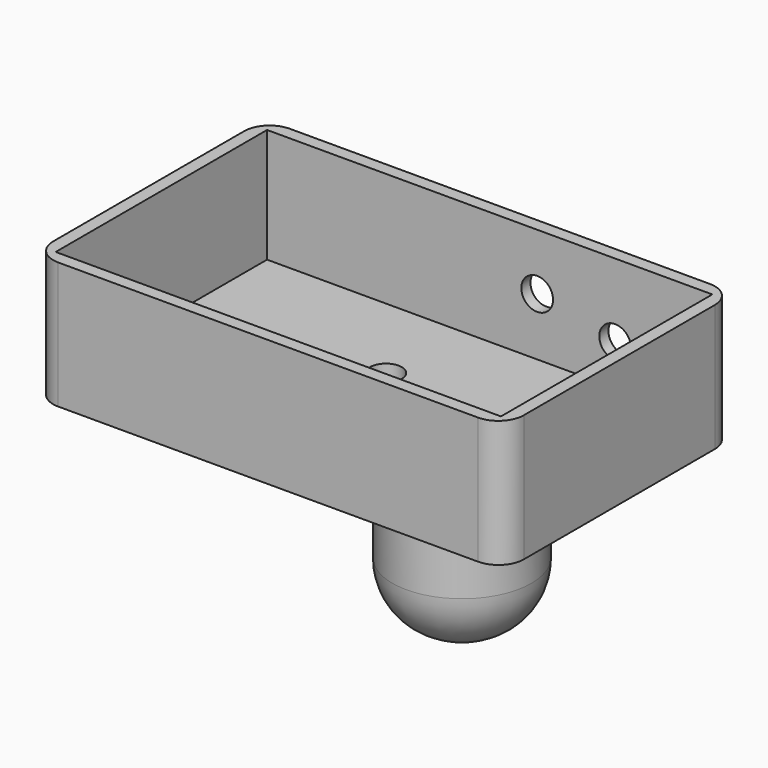
from build123d import *

# Parameters (mm, degrees)
F0_W           = 94.2332278937
F0_H           = 57.9777825624
F1_DEPTH       = 25.4
F2_T           = -2.54
F3_R           = 5.08
F5_D           = 6.35
F7_D           = 6.35
F7_DEPTH       = 12.7
F7_CBORE_D     = 12.7
F7_CBORE_DEPTH = 0.254
F7_TIP         = 1.9077324654
F9_D           = 6.35
F9_DEPTH       = 12.7
F9_CBORE_D     = 12.7
F9_CBORE_DEPTH = 0.254
F9_TIP         = 1.9077324654
F10_R          = 13.9169366501
F11_DEPTH      = 25.4
F12_R          = 12.7
F13_W          = 27.7714207768
F13_H          = 7.534484379
F14_DEPTH      = 25.4
F15_R          = 12.7
F16_T1_DEPTH   = 12.7
F16_T3_DEPTH   = 2.3714207768
F16_T6_ANGLE   = 90
F16_T8_ANGLE   = 90
F16_T10_ANGLE  = 90
F16_T12_ANGLE  = 90


# Not quite as in the source:
# - a fillet or chamfer that OpenCascade refuses, or shapes differently, is made with other operations: its cross-section is extruded or revolved along the edge and cut away or added


with BuildPart() as f1:
    # F0 (on Top) → F1 (new body)
    with BuildSketch(Plane.XY):
        with Locations((-38.147569634, 3.4275231883)):
            Rectangle(F0_W, F0_H)
    extrude(amount=F1_DEPTH)

    # F2
    f2_openings = [f1.faces().sort_by_distance(p)[0] for p in [
        (-38.14757, 3.427523, 25.4),
    ]]
    offset(amount=F2_T, openings=f2_openings)

    # F3
    f3_edges = [f1.edges().sort_by_distance(p)[0] for p in [
        (-85.264184, -25.561368, 12.7),
        (8.969044, -25.561368, 12.7),
        (8.969044, 32.416414, 12.7),
        (-85.264184, 32.416414, 12.7),
    ]]
    fillet(f3_edges, radius=F3_R)

    # F5 (through all)
    with Locations(Plane.XY.offset(2.54)):
        with Locations((-44.2425459623, 11.5331579)):
            Hole(F5_D / 2)

    # F7
    with Locations(Plane.XY.offset(2.54)):
        with Locations((-63.0617812276, -7.2897328064)):
            CounterBoreHole(F7_D / 2, F7_CBORE_D / 2, F7_CBORE_DEPTH, depth=F7_DEPTH)
            with Locations((0, 0, -(F7_DEPTH + F7_TIP / 2))):  # 118° drill point
                Cone(0, F7_D / 2, F7_TIP, mode=Mode.SUBTRACT)

    # F9
    with Locations(Plane(origin=(0, 32.4164144695, 0), x_dir=(-1, 0, 0), z_dir=(0, 1, 0))):
        with Locations((13.0262067541, 10.6704961509), (28.6341179162, 14.0921706334)):
            CounterBoreHole(F9_D / 2, F9_CBORE_D / 2, F9_CBORE_DEPTH, depth=F9_DEPTH)
            with Locations((0, 0, -(F9_DEPTH + F9_TIP / 2))):  # 118° drill point
                Cone(0, F9_D / 2, F9_TIP, mode=Mode.SUBTRACT)

    # F10 (on face) → F11 (join)
    with BuildSketch(Plane(origin=(0, 0, 0), x_dir=(1, 0, 0), z_dir=(0, 0, -1))):
        with Locations((-14.1745125875, 7.0280302316)):
            Circle(F10_R)
    extrude(amount=F11_DEPTH)

    # F12
    f12_edges = [f1.edges().sort_by_distance(p)[0] for p in [
        (-28.091449, -7.02803, -25.4),
    ]]
    fillet(f12_edges, radius=F12_R)

    # F13 (on face) → F14 (join)
    with BuildSketch(Plane(origin=(0, 0, 0), x_dir=(1, 0, 0), z_dir=(0, 0, -1))):
        with Locations((-67.7874796093, -15.7441017218)):
            Rectangle(F13_W, F13_H)
    extrude(amount=F14_DEPTH)

    # F15
    f15_edges = [f1.edges().sort_by_distance(p)[0] for p in [
        (-53.901769, 15.744102, -25.4),
        (-81.67319, 15.744102, -25.4),
    ]]
    fillet(f15_edges, radius=F15_R)

    # F16: fillet of radius 5.08 on 2 edges, made by hand

    # F16_s2 → F16_t1 (cut)
    with BuildSketch(Plane.XY.offset(-12.7)):
        with BuildLine():
            ThreePointArc((-58.9817692208, 19.5113439113), (-55.3896667724, 18.0234463597), (-53.9017692208, 14.4313439113))
            Line((-53.9017692208, 14.4313439113), (-53.9017692208, 19.5113439113))
            Line((-53.9017692208, 19.5113439113), (-58.9817692208, 19.5113439113))
        make_face()
        with BuildLine():
            ThreePointArc((-81.6731899977, 14.4313439113), (-80.1852924461, 18.0234463597), (-76.5931899977, 19.5113439113))
            Line((-76.5931899977, 19.5113439113), (-81.6731899977, 19.5113439113))
            Line((-81.6731899977, 19.5113439113), (-81.6731899977, 14.4313439113))
        make_face()
        with BuildLine():
            ThreePointArc((-81.6731899977, 17.0568595323), (-80.1852924461, 13.4647570839), (-76.5931899977, 11.9768595323))
            Line((-76.5931899977, 11.9768595323), (-81.6731899977, 11.9768595323))
            Line((-81.6731899977, 11.9768595323), (-81.6731899977, 17.0568595323))
        make_face()
        with BuildLine():
            ThreePointArc((-58.9817692208, 11.9768595323), (-55.3896667724, 13.4647570839), (-53.9017692208, 17.0568595323))
            Line((-53.9017692208, 17.0568595323), (-53.9017692208, 11.9768595323))
            Line((-53.9017692208, 11.9768595323), (-58.9817692208, 11.9768595323))
        make_face()
    extrude(amount=F16_T1_DEPTH, mode=Mode.SUBTRACT)

    # F16_s4 → F16_t3 (cut)
    with BuildSketch(Plane.YZ.offset(-68.9731899977)):
        with BuildLine():
            ThreePointArc((19.5113439113, -20.32), (18.0234463597, -23.9121024484), (14.4313439113, -25.4))
            Line((14.4313439113, -25.4), (19.5113439113, -25.4))
            Line((19.5113439113, -25.4), (19.5113439113, -20.32))
        make_face()
        with BuildLine():
            ThreePointArc((11.9768595323, -20.32), (13.4647570839, -23.9121024484), (17.0568595323, -25.4))
            Line((17.0568595323, -25.4), (11.9768595323, -25.4))
            Line((11.9768595323, -25.4), (11.9768595323, -20.32))
        make_face()
    extrude(amount=F16_T3_DEPTH, mode=Mode.SUBTRACT)

    # F16_s5 → F16_t6 (revolve, cut)
    with BuildSketch(Plane.XY.offset(-12.7)):
        with BuildLine():
            ThreePointArc((-76.5931899977, 11.9768595323), (-80.1852924461, 13.4647570839), (-81.6731899977, 17.0568595323))
            Line((-81.6731899977, 17.0568595323), (-81.6731899977, 11.9768595323))
            Line((-81.6731899977, 11.9768595323), (-76.5931899977, 11.9768595323))
        make_face()
    revolve(axis=Axis((-68.9731899977, 11.9768595323, -12.7), (0, -1, 0)), revolution_arc=F16_T6_ANGLE, mode=Mode.SUBTRACT)

    # F16_s7 → F16_t8 (revolve, cut)
    with BuildSketch(Plane.XY.offset(-12.7)):
        with BuildLine():
            ThreePointArc((-58.9817692208, 19.5113439113), (-55.3896667724, 18.0234463597), (-53.9017692208, 14.4313439113))
            Line((-53.9017692208, 14.4313439113), (-53.9017692208, 19.5113439113))
            Line((-53.9017692208, 19.5113439113), (-58.9817692208, 19.5113439113))
        make_face()
    revolve(axis=Axis((-66.6017692208, 19.5113439113, -12.7), (0, 1, 0)), revolution_arc=F16_T8_ANGLE, mode=Mode.SUBTRACT)

    # F16_s9 → F16_t10 (revolve, cut)
    with BuildSketch(Plane.XY.offset(-12.7)):
        with BuildLine():
            ThreePointArc((-81.6731899977, 14.4313439113), (-80.1852924461, 18.0234463597), (-76.5931899977, 19.5113439113))
            Line((-76.5931899977, 19.5113439113), (-81.6731899977, 19.5113439113))
            Line((-81.6731899977, 19.5113439113), (-81.6731899977, 14.4313439113))
        make_face()
    revolve(axis=Axis((-68.9731899977, 19.5113439113, -12.7), (0, -1, 0)), revolution_arc=F16_T10_ANGLE, mode=Mode.SUBTRACT)

    # F16_s11 → F16_t12 (revolve, cut)
    with BuildSketch(Plane.XY.offset(-12.7)):
        with BuildLine():
            ThreePointArc((-58.9817692208, 11.9768595323), (-55.3896667724, 13.4647570839), (-53.9017692208, 17.0568595323))
            Line((-53.9017692208, 17.0568595323), (-53.9017692208, 11.9768595323))
            Line((-53.9017692208, 11.9768595323), (-58.9817692208, 11.9768595323))
        make_face()
    revolve(axis=Axis((-66.6017692208, 11.9768595323, -12.7), (0, 1, 0)), revolution_arc=F16_T12_ANGLE, mode=Mode.SUBTRACT)


solid = f1.part
